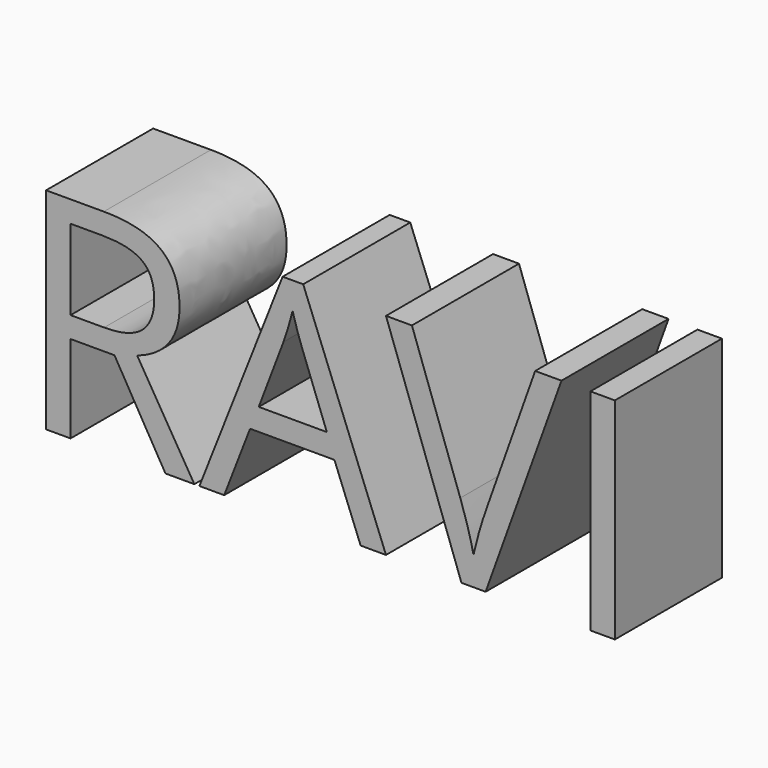
from build123d import *

# Parameters (mm, degrees)
F0_TEXT_SIZE = 11.016190466
F1_DEPTH     = 5


# Not quite as in the source:
# - Text() gives the source's letters only with a copy of the font that has no kerning and outlines rounded to 1/6400 em; it was checked with that copy


with BuildPart() as f1:
    # F0 (on Front) → F1 (new body)
    with BuildSketch(Plane.XZ):
        with Locations((-12.0391221717, -4.1074648034)):
            Text('RAVI', F0_TEXT_SIZE, font='Open Sans', text_align=(TextAlign.LEFT, TextAlign.BOTTOM))
    extrude(amount=F1_DEPTH)


solid = f1.part
